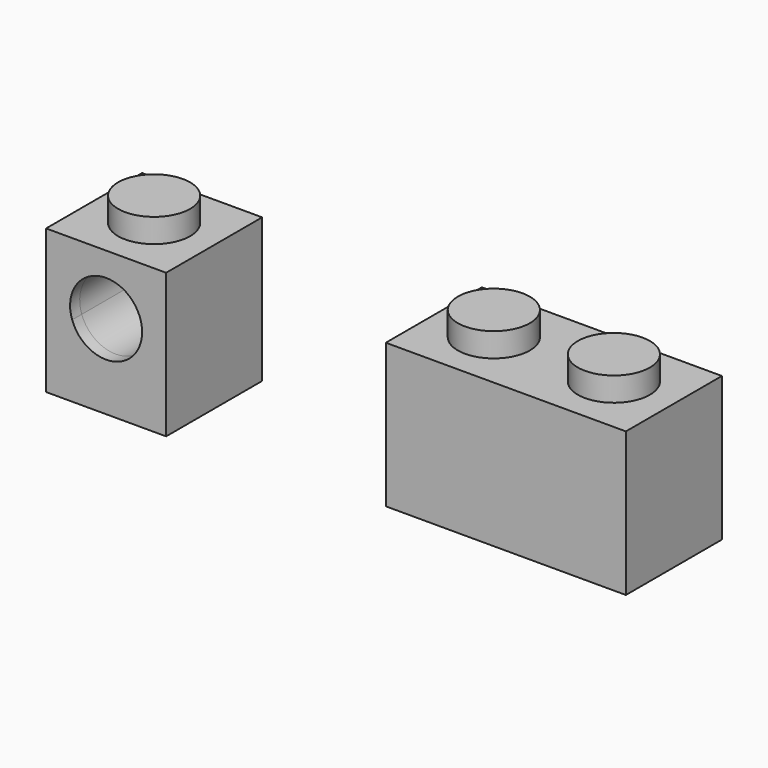
from build123d import *
from build123d import SkipClean  # not in build123d's __all__

# Parameters (mm, degrees)
F0_W      = 40
F0_H      = 20
F1_DEPTH  = 24
F2_R      = 6
F3_DEPTH  = 4
F4_W      = 18
F4_H      = 8
F5_DEPTH  = 22
F6_R      = 5
F7_DEPTH  = 4
F9_DEPTH  = 22
F10_R     = 2
F11_DEPTH = 22
F12_W     = 20
F12_H     = 20
F13_DEPTH = 24
F15_DEPTH = 4
F16_W     = 8
F16_H     = 8
F17_DEPTH = 22
F19_DEPTH = 20
F20_DEPTH = 25


with BuildPart() as f1:
    # F0 (on Top) → F1 (new body)
    with BuildSketch(Plane.XY):
        with Locations((-104.0465351939, -69.9002796412)):
            Rectangle(F0_W, F0_H)
    extrude(amount=F1_DEPTH)

    # F2 (on face) → F3 (join)
    with BuildSketch(Plane.XY.offset(24)):
        with BuildLine():
            ThreePointArc((-120.0465351939, -69.9002796412), (-114.0465351939, -75.9002796412), (-108.0465351939, -69.9002796412))
            ThreePointArc((-108.0465351939, -69.9002796412), (-114.0465351939, -63.9002796412), (-120.0465351939, -69.9002796412))
        make_face()
        with Locations((-94.0465351939, -69.9002796412)):
            Circle(F2_R)
    extrude(amount=F3_DEPTH)

    # F4 (on face) → F5 (cut)
    with BuildSketch(Plane(origin=(0, 0, 0), x_dir=(1, 0, 0), z_dir=(0, 0, -1))):
        with Locations((-113.0465351939, 73.9002796412)):
            Rectangle(F4_W, F4_H)
        with Locations((-113.0465351939, 65.9002796412)):
            Rectangle(F4_W, F4_H)
        with Locations((-95.0465351939, 65.9002796412)):
            Rectangle(F4_W, F4_H)
        with Locations((-95.0465351939, 73.9002796412)):
            Rectangle(F4_W, F4_H)
    extrude(amount=-F5_DEPTH, mode=Mode.SUBTRACT)

    # F6 (on face) → F7 (cut)
    with BuildSketch(Plane(origin=(0, 0, 22), x_dir=(1, 0, 0), z_dir=(0, 0, -1))):
        with Locations((-94.0465351939, 69.9002796412)):
            Circle(F6_R)
        with BuildLine():
            ThreePointArc((-109.0465351939, 69.9002796412), (-114.0465351939, 74.9002796412), (-119.0465351939, 69.9002796412))
            ThreePointArc((-119.0465351939, 69.9002796412), (-114.0465351939, 64.9002796412), (-109.0465351939, 69.9002796412))
        make_face()
    extrude(amount=-F7_DEPTH, mode=Mode.SUBTRACT)

    # F8 (on face) → F9 (join)
    with BuildSketch(Plane(origin=(0, 0, 22), x_dir=(1, 0, 0), z_dir=(0, 0, -1))):
        with BuildLine():
            ThreePointArc((-107.0465351939, 69.9002796412), (-104.0465351939, 66.9002796412), (-101.0465351939, 69.9002796412))
            ThreePointArc((-101.0465351939, 69.9002796412), (-104.0465351939, 72.9002796412), (-107.0465351939, 69.9002796412))
        make_face()
    extrude(amount=F9_DEPTH)

    # F10 (on face) → F11 (cut)
    with BuildSketch(Plane(origin=(0, 0, 0), x_dir=(1, 0, 0), z_dir=(0, 0, -1))):
        with Locations((-104.0465351939, 69.9002796412)):
            Circle(F10_R)
    extrude(amount=-F11_DEPTH, mode=Mode.SUBTRACT)


with BuildPart() as f13:
    # F12 (on Top) → F13 (new body)
    with BuildSketch(Plane.XY):
        with Locations((-168.6746275425, -72.3669731617)):
            Rectangle(F12_W, F12_H)
    extrude(amount=F13_DEPTH)

    # F14 (on face) → F15 (join)
    with BuildSketch(Plane.XY.offset(24)):
        with BuildLine():
            ThreePointArc((-162.6746275425, -72.3669731617), (-168.6746275425, -66.3669731617), (-174.6746275425, -72.3669731617))
            ThreePointArc((-174.6746275425, -72.3669731617), (-168.6746275425, -78.3669731617), (-162.6746275425, -72.3669731617))
        make_face()
    extrude(amount=F15_DEPTH)

    # F16 (on face) → F17 (cut)
    with BuildSketch(Plane(origin=(0, 0, 0), x_dir=(1, 0, 0), z_dir=(0, 0, -1))):
        with Locations((-172.6746275425, 76.3669731617)):
            Rectangle(F16_W, F16_H)
        with Locations((-172.6746275425, 68.3669731617)):
            Rectangle(F16_W, F16_H)
        with Locations((-164.6746275425, 76.3669731617)):
            Rectangle(F16_W, F16_H)
        with Locations((-164.6746275425, 68.3669731617)):
            Rectangle(F16_W, F16_H)
    extrude(amount=-F17_DEPTH, mode=Mode.SUBTRACT)

    # F18 (on face) → F19 (join)
    with BuildSketch(Plane.XZ.offset(82.3669731617)):
        with BuildLine():
            Line((-174.331481792, 12), (-175.382831475, 12))
            ThreePointArc((-175.382831475, 12), (-168.6746275425, 7), (-161.96642361, 12))
            Line((-161.96642361, 12), (-163.017773293, 12))
            ThreePointArc((-163.017773293, 12), (-168.6746275425, 8), (-174.331481792, 12))
        make_face()
        with BuildLine():
            ThreePointArc((-161.6746275425, 14), (-169.6852146175, 20.9266668581), (-175.382831475, 12))
            Line((-175.382831475, 12), (-174.331481792, 12))
            ThreePointArc((-174.331481792, 12), (-169.6892394149, 19.9135913579), (-162.6746275425, 14))
            ThreePointArc((-162.6746275425, 14), (-162.7610361846, 12.9853881276), (-163.017773293, 12))
            Line((-163.017773293, 12), (-161.96642361, 12))
            ThreePointArc((-161.96642361, 12), (-161.7479606843, 12.989412925), (-161.6746275425, 14))
        make_face()
    extrude(amount=-F19_DEPTH)

    # F18 (on face) → F20 (cut)
    with BuildSketch(Plane.XZ.offset(82.3669731617)):
        with BuildLine():
            ThreePointArc((-162.6746275425, 14), (-169.6892394149, 19.9135913579), (-174.331481792, 12))
            Line((-174.331481792, 12), (-168.6746275425, 12))
            Line((-168.6746275425, 12), (-163.017773293, 12))
            ThreePointArc((-163.017773293, 12), (-162.7610361846, 12.9853881276), (-162.6746275425, 14))
        make_face()
        with BuildLine():
            Line((-168.6746275425, 12), (-174.331481792, 12))
            ThreePointArc((-174.331481792, 12), (-168.6746275425, 8), (-163.017773293, 12))
            Line((-163.017773293, 12), (-168.6746275425, 12))
        make_face()
    with SkipClean():  # cleaning this boolean's faces spoils the solid; the shape is the same uncleaned
        extrude(amount=-F20_DEPTH, mode=Mode.SUBTRACT)


solid = Compound([f1.part, f13.part])
